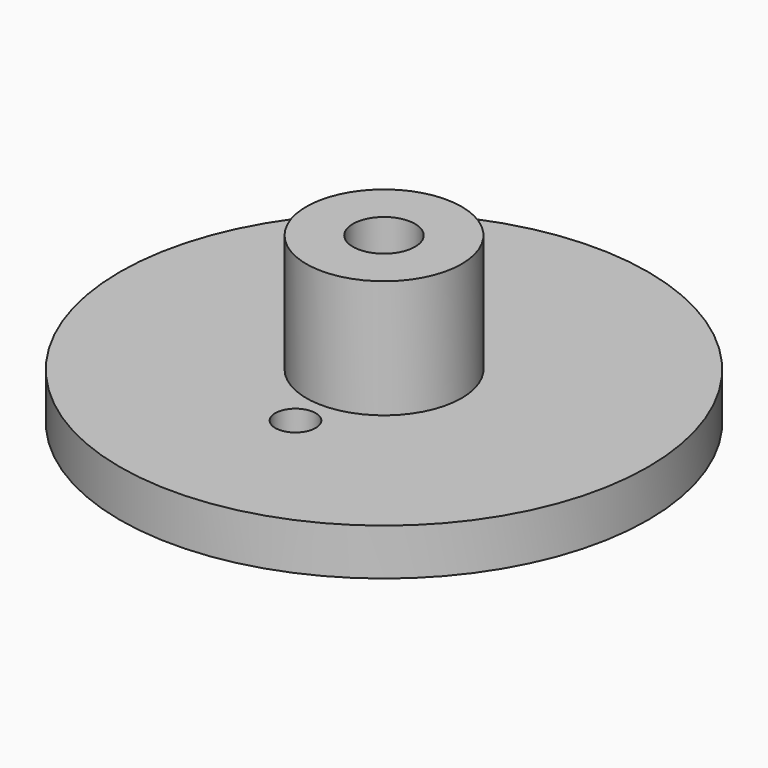
from build123d import *

# Parameters (mm, degrees)
F0_R     = 8.5
F0_R_2   = 1
F1_DEPTH = 1.5
F2_R     = 2.5
F2_R_2   = 1
F3_DEPTH = 3.8
F4_R     = 0.6498381819
F5_DEPTH = 1.5


# Not quite as in the source:
# - a feature names something its author has since deleted; it is built from what else it names


with BuildPart() as f1:
    # F0 (on Top) → F1 (new body)
    with BuildSketch(Plane.XY):
        Circle(F0_R)
        Circle(F0_R_2, mode=Mode.SUBTRACT)
    extrude(amount=F1_DEPTH)

    # F2 (on face) → F3 (join)
    with BuildSketch(Plane.XY.offset(1.5)):
        Circle(F2_R)
        Circle(F2_R_2, mode=Mode.SUBTRACT)
    extrude(amount=F3_DEPTH)

    # F4 (on Top) → F5 (cut, through all)
    with BuildSketch(Plane.XY):
        with Locations((0, -3.5616646055)):
            Circle(F4_R)
    extrude(amount=F5_DEPTH, mode=Mode.SUBTRACT)


solid = f1.part
